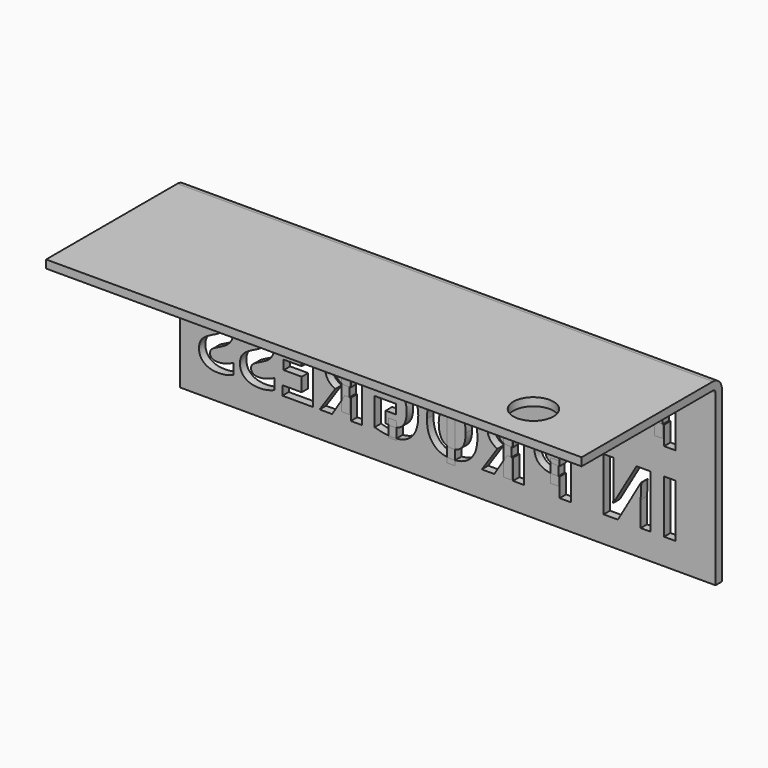
from build123d import *

# Parameters (mm, degrees)
F1_DEPTH     = 80
F2_R         = 0.5
F3_R         = 1.7
F4_R         = 3
F5_DEPTH     = 1.201
F6_TEXT_SIZE = 11.1111111111
F7_DEPTH     = 25
F8_W         = 1.2
F8_H         = 4.2865481228
F8_H_2       = 4.1067898273
F8_H_3       = 2.8988959385
F8_H_4       = 3.3590332605
F8_H_5       = 5.2742045373
F8_H_6       = 9.6258225385
F8_H_7       = 4.3492270634
F8_H_8       = 2.576212341
F9_DEPTH     = 1.2


# Not quite as in the source:
# - Text() gives the source's letters only with a copy of the font that has no kerning and outlines rounded to 1/6400 em; it was checked with that copy


with BuildPart() as f1:
    # F0 (on Right) → F1 (new body)
    with BuildSketch(Plane.YZ):
        Polygon((0, 25.8), (0, 0), (1.2, 0), (1.2, 27), (-25, 27), (-25, 25.8), align=None)
    extrude(amount=-F1_DEPTH)

    # F2
    f2_edges = [f1.edges().sort_by_distance(p)[0] for p in [
        (-40, 0, 25.8),
    ]]
    fillet(f2_edges, radius=F2_R)

    # F3
    f3_edges = [f1.edges().sort_by_distance(p)[0] for p in [
        (-40, 1.2, 27),
    ]]
    fillet(f3_edges, radius=F3_R)

    # F4 (on face) → F5 (cut, through all)
    with BuildSketch(Plane(origin=(0, 0, 25.8), x_dir=(1, 0, 0), z_dir=(0, 0, -1))):
        with Locations((-12, 19)):
            Circle(F4_R)
    extrude(amount=-F5_DEPTH, mode=Mode.SUBTRACT)

    # F6 (on face) → F7 (cut)
    with BuildSketch(Plane(origin=(0, 1.2, 0), x_dir=(-1, 0, 0), z_dir=(0, 1, 0))):
        with Locations((5, 15.8)):
            Text('PRINTING', F6_TEXT_SIZE, font='Open Sans', font_style=FontStyle.BOLD, text_align=(TextAlign.LEFT, TextAlign.BOTTOM))
        with Locations((5, 3.8928682059)):
            Text('IN PROGRESS', F6_TEXT_SIZE, font='Open Sans', font_style=FontStyle.BOLD, text_align=(TextAlign.LEFT, TextAlign.BOTTOM))
    extrude(amount=-F7_DEPTH, mode=Mode.SUBTRACT)

    # F8 (on face) → F9 (join, through all)
    with BuildSketch(Plane(origin=(0, 1.2, 0), x_dir=(-1, 0, 0), z_dir=(0, 1, 0))):
        with Locations((8.4805555556, 18.8764380291)):
            Rectangle(F8_W, F8_H)
        with Locations((15.4579861111, 19.2113500088)):
            Rectangle(F8_W, F8_H_2)
        with Locations((55.6822916667, 16.2169775867)):
            Rectangle(F8_W, F8_H_3)
        with Locations((24.0795138889, 7.0917455014)):
            Rectangle(F8_W, F8_H_4)
        with Locations((31.0569444444, 6.5730586648)):
            Rectangle(F8_W, F8_H_5)
        with Locations((39.4971882045, 7.8792040003)):
            Rectangle(F8_W, F8_H_6)
        with Locations((55.2809027778, 6.8517127074)):
            Rectangle(F8_W, F8_H_7)
        with Locations((48.2673611111, 4.8313245354)):
            Rectangle(F8_W, F8_H_8)
    extrude(amount=-F9_DEPTH)


solid = f1.part
